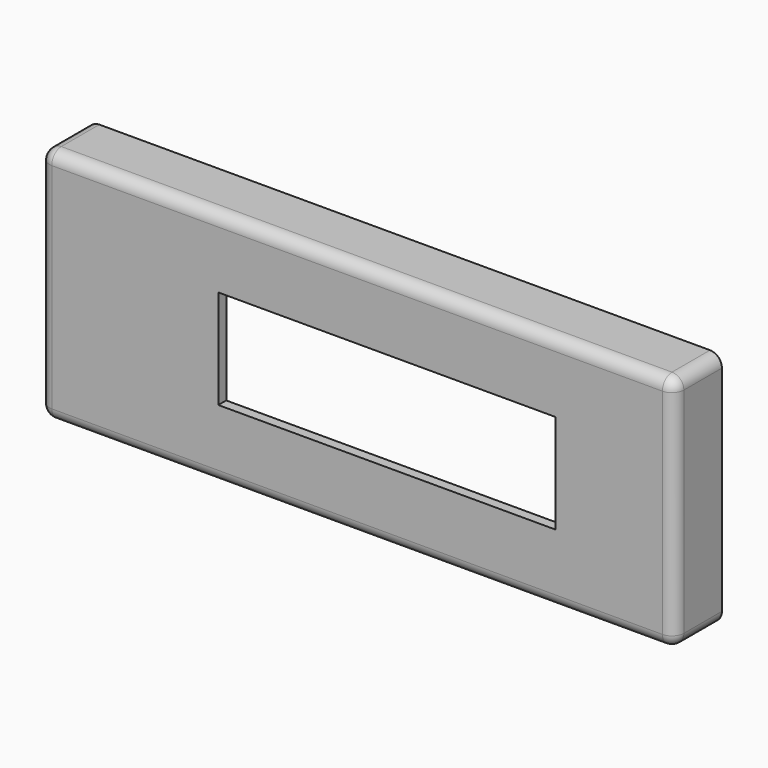
from build123d import *

# Parameters (mm, degrees)
F0_W     = 160
F0_H     = 60
F1_DEPTH = 15
F2_R     = 3
F3_T     = -2.5
F5_DEPTH = 10
F6_W     = 85
F6_H     = 25
F7_DEPTH = 25


with BuildPart() as f1:
    # F0 (on Front) → F1 (new body)
    with BuildSketch(Plane.XZ):
        with Locations((80, 30)):
            Rectangle(F0_W, F0_H)
    extrude(amount=F1_DEPTH)

    # F2
    f2_edges = [f1.edges().sort_by_distance(p)[0] for p in [
        (0, -7.5, 60),
        (80, -15, 60),
        (0, -15, 30),
        (80, -15, 0),
        (0, -7.5, 0),
        (160, -7.5, 0),
        (160, -7.5, 60),
        (160, -15, 30),
    ]]
    fillet(f2_edges, radius=F2_R)

    # F3
    f3_openings = [f1.faces().sort_by_distance(p)[0] for p in [
        (80, 0, 30),
    ]]
    offset(amount=F3_T, openings=f3_openings)

    # F4 (on face) → F5 (join)
    with BuildSketch(Plane(origin=(0, -12.5, 0), x_dir=(-1, 0, 0), z_dir=(0, 1, 0))):
        with BuildLine():
            ThreePointArc((-157, 50.417424305), (-152.2613872125, 50.8166998673), (-150, 55))
            ThreePointArc((-150, 55), (-150.1054684353, 56.0215482184), (-150.417424305, 57))
            Line((-150.417424305, 57), (-157, 57))
            Line((-157, 57), (-157, 50.417424305))
        make_face()
        with BuildLine():
            Line((-3, 57), (-9.582575695, 57))
            ThreePointArc((-9.582575695, 57), (-8.5355339059, 51.4644660941), (-3, 50.417424305))
            Line((-3, 50.417424305), (-3, 57))
        make_face()
        with BuildLine():
            ThreePointArc((-150, 5), (-152.2613872125, 9.1833001327), (-157, 9.582575695))
            Line((-157, 9.582575695), (-157, 3))
            Line((-157, 3), (-150.417424305, 3))
            ThreePointArc((-150.417424305, 3), (-150.1054684353, 3.9784517816), (-150, 5))
        make_face()
        with BuildLine():
            Line((-3, 3), (-3, 9.582575695))
            ThreePointArc((-3, 9.582575695), (-8.5355339059, 8.5355339059), (-9.582575695, 3))
            Line((-9.582575695, 3), (-3, 3))
        make_face()
    extrude(amount=F5_DEPTH)

    # F6 (on face) → F7 (cut)
    with BuildSketch(Plane(origin=(0, -12.5, 0), x_dir=(-1, 0, 0), z_dir=(0, 1, 0))):
        with Locations((-87.5, 30)):
            Rectangle(F6_W, F6_H)
    extrude(amount=-F7_DEPTH, mode=Mode.SUBTRACT)


solid = f1.part
